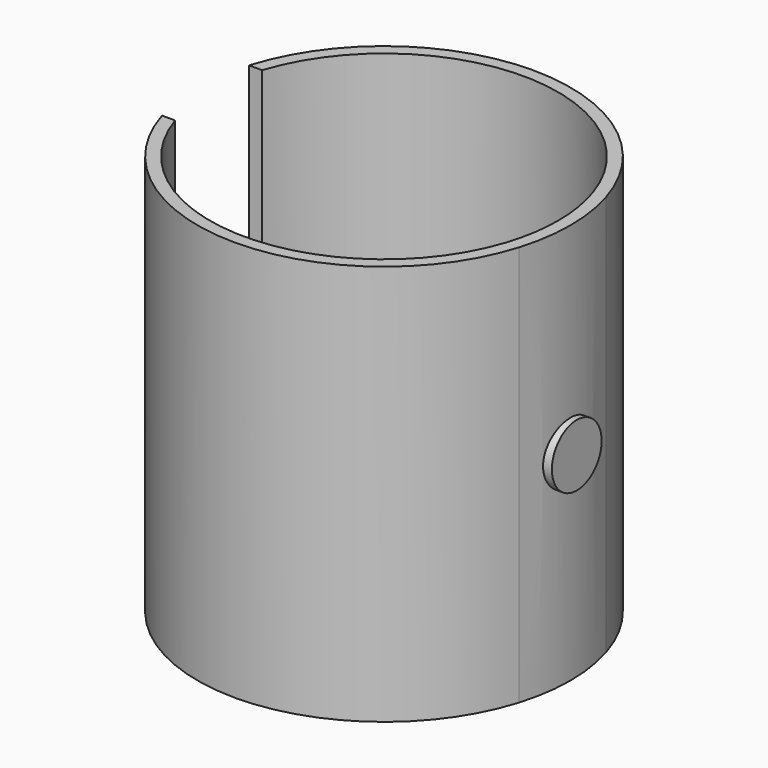
from build123d import *

# Parameters (mm, degrees)
F1_DEPTH = 81.8546242
F2_R     = 6.35
F3_DEPTH = 39.37
F4_R     = 35.56
F5_DEPTH = 107.95


# Not quite as in the source:
# - a feature names something its author has since deleted; it is built from what else it names


with BuildPart() as f1:
    # F0 (on Top) → F1 (new body)
    with BuildSketch(Plane.XY):
        with BuildLine():
            Line((33.7800627271, 11.1094987354), (36.4443279242, 11.1094987354))
            ThreePointArc((36.4443279242, 11.1094987354), (0, 38.1), (-36.4443279242, 11.1094987354))
            Line((-36.4443279242, 11.1094987354), (-33.7800627271, 11.1094987354))
            ThreePointArc((-33.7800627271, 11.1094987354), (0, 35.56), (33.7800627271, 11.1094987354))
        make_face()
        with BuildLine():
            ThreePointArc((-36.4443279242, -11.1094987354), (0, -38.1), (36.4443279242, -11.1094987354))
            Line((36.4443279242, -11.1094987354), (33.7800627271, -11.1094987354))
            ThreePointArc((33.7800627271, -11.1094987354), (0, -35.56), (-33.7800627271, -11.1094987354))
            Line((-33.7800627271, -11.1094987354), (-36.4443279242, -11.1094987354))
        make_face()
        with BuildLine():
            Line((36.4443279242, -11.1094987354), (36.4443279242, 11.1094987354))
            Line((36.4443279242, 11.1094987354), (33.7800627271, 11.1094987354))
            ThreePointArc((33.7800627271, 11.1094987354), (35.1121961046, 5.6255919433), (35.56, 0))
            ThreePointArc((35.56, 0), (35.1121961046, -5.6255919433), (33.7800627271, -11.1094987354))
            Line((33.7800627271, -11.1094987354), (36.4443279242, -11.1094987354))
        make_face()
        with BuildLine():
            ThreePointArc((36.4443279242, -11.1094987354), (37.683808817, -5.6160976704), (38.1, 0))
            ThreePointArc((38.1, 0), (37.683808817, 5.6160976704), (36.4443279242, 11.1094987354))
            Line((36.4443279242, 11.1094987354), (36.4443279242, -11.1094987354))
        make_face()
    extrude(amount=F1_DEPTH)

    # F2 (on Right) → F3 (join)
    with BuildSketch(Plane.YZ):
        with Locations((0, 40.9273121)):
            Circle(F2_R)
    extrude(amount=F3_DEPTH)

    # F4 (on Top) → F5 (cut, symmetric)
    with BuildSketch(Plane.XY):
        Circle(F4_R)
    extrude(amount=F5_DEPTH, both=True, mode=Mode.SUBTRACT)


solid = f1.part
